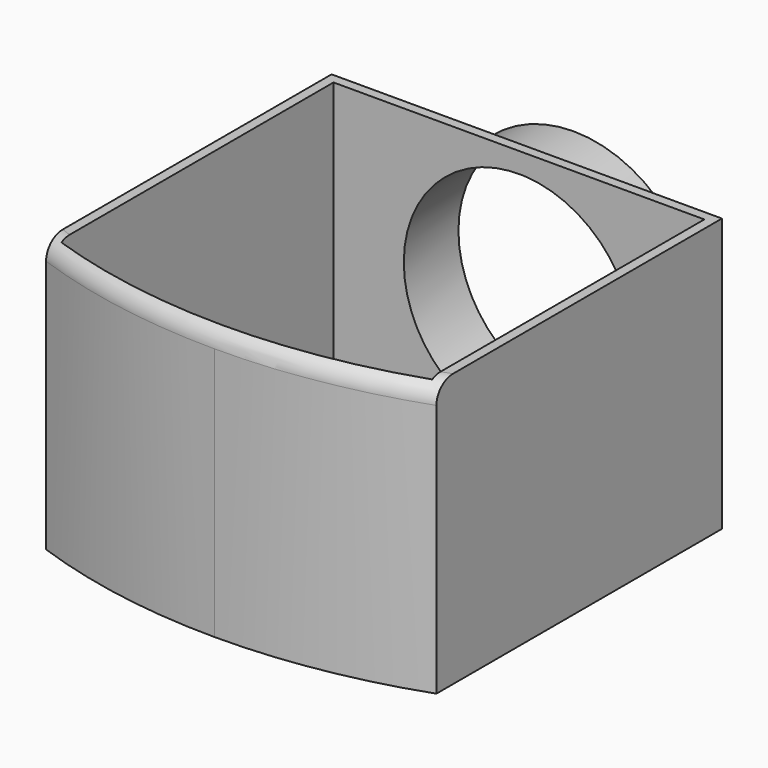
from build123d import *

# Parameters (mm, degrees)
F1_DEPTH    = 70
F2_T        = -2.5
F3_T2_ANGLE = 48.492455887
F5_DEPTH    = 15
F6_T        = -2.5
F7_DEPTH    = 25


# Not quite as in the source:
# - a fillet or chamfer that OpenCascade refuses, or shapes differently, is made with other operations: its cross-section is extruded or revolved along the edge and cut away or added


with BuildPart() as f1:
    # F0 (on Top) → F1 (new body)
    with BuildSketch(Plane.XY):
        with BuildLine():
            ThreePointArc((-50, -141.4213562373), (-25.3652968089, -147.839783948), (0, -150))
            ThreePointArc((0, -150), (25.3652968089, -147.839783948), (50, -141.4213562373))
            Line((50, -141.4213562373), (50, -50))
            Line((50, -50), (0, -50))
            Line((0, -50), (-50, -50))
            Line((-50, -50), (-50, -141.4213562373))
        make_face()
    extrude(amount=F1_DEPTH)

    # F2
    f2_openings = [f1.faces().sort_by_distance(p)[0] for p in [
        (0, -98.620362, 70),
    ]]
    offset(amount=F2_T, openings=f2_openings)

    # F3: fillet of radius 5 on 1 edges, made by hand

    # F3_s1 → F3_t2 (revolve, cut)
    with BuildSketch(Plane(origin=(0, 0, 0), x_dir=(0, 0, 1), z_dir=(0.9117890812, 0.410658826, 0))):
        with BuildLine():
            ThreePointArc((65, 150), (68.5355339059, 148.5355339059), (70, 145))
            Line((70, 145), (70, 150))
            Line((70, 150), (65, 150))
        make_face()
    revolve(axis=Axis((0, 0, 70), (0, 0, -1)), revolution_arc=F3_T2_ANGLE, mode=Mode.SUBTRACT)

    # F4 (on face) → F5 (join)
    with BuildSketch(Plane(origin=(0, -50, 0), x_dir=(-1, 0, 0), z_dir=(0, 1, 0))):
        with BuildLine():
            ThreePointArc((32, 35.3235527873), (-22.627416998, 57.9509697853), (0, 3.3235527873))
            ThreePointArc((0, 3.3235527873), (22.627416998, 12.6961357893), (32, 35.3235527873))
        make_face()
    extrude(amount=F5_DEPTH)

    # F6
    f6_openings = [f1.faces().sort_by_distance(p)[0] for p in [
        (0, -35, 35.323553),
    ]]
    offset(amount=F6_T, openings=f6_openings, kind=Kind.INTERSECTION)

    # F7 (cut): a face of the model
    f7_faces = [f1.faces().sort_by_distance(p)[0] for p in [
        (0, -50, 35.3235527873),
    ]]
    extrude(f7_faces, amount=-F7_DEPTH, mode=Mode.SUBTRACT)


solid = f1.part
